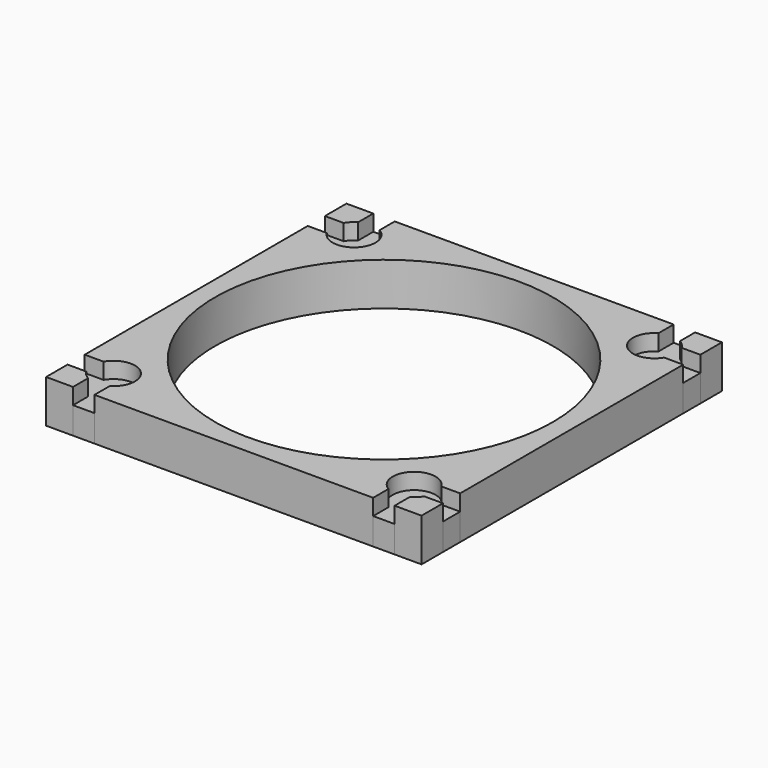
from build123d import *

# Parameters (mm, degrees)
F0_R     = 31.5
F1_DEPTH = 8
F3_DEPTH = 8
F4_DEPTH = 5
F5_DEPTH = 8
F6_DEPTH = 5


# Not quite as in the source:
# - a feature names something its author has since deleted; it is built from what else it names


with BuildPart() as f1:
    # F0 (on Top) → F1 (new body)
    with BuildSketch(Plane.XY):
        with BuildLine():
            Line((-31.4370289465, 25.9772784561), (-35, 25.9772784561))
            Line((-35, 25.9772784561), (-35, -26))
            Line((-35, -26), (-31.4875550445, -26))
            ThreePointArc((-31.4875550445, -26), (-25.2140139956, -25.1527118045), (-25.9772784561, -31.4370289465))
            Line((-25.9772784561, -31.4370289465), (-25.9772784561, -35))
            Line((-25.9772784561, -35), (25.9772784561, -35))
            Line((25.9772784561, -35), (25.9772784561, -31.4370289465))
            ThreePointArc((25.9772784561, -31.4370289465), (25.2140139956, -25.1527118045), (31.4875550445, -26))
            Line((31.4875550445, -26), (35, -26))
            Line((35, -26), (35, -25.5))
            Line((35, -25.5), (35, 25.9772784561))
            Line((35, 25.9772784561), (31.4370289465, 25.9772784561))
            ThreePointArc((31.4370289465, 25.9772784561), (25.1527118045, 25.2140139956), (26, 31.4875550445))
            Line((26, 31.4875550445), (26, 35))
            Line((26, 35), (-25.5, 35))
            Line((-25.5, 35), (-26, 35))
            Line((-26, 35), (-26, 31.4875550445))
            ThreePointArc((-26, 31.4875550445), (-25.1527118045, 25.2140139956), (-31.4370289465, 25.9772784561))
        make_face()
        Circle(F0_R, mode=Mode.SUBTRACT)
    extrude(amount=F1_DEPTH)


with BuildPart() as f3:
    # F0 (on Top) → F3 (new body)
    with BuildSketch(Plane.XY):
        with BuildLine():
            Line((-31.9894003868, 35), (-35, 35))
            Line((-35, 35), (-35, 29.9772784561))
            Line((-35, 29.9772784561), (-31.4903535301, 29.9772784561))
            ThreePointArc((-31.4903535301, 29.9772784561), (-30.8471440629, 30.83303893), (-30, 31.4875550445))
            Line((-30, 31.4875550445), (-30, 35))
            Line((-30, 35), (-30.5, 35))
            Line((-30.5, 35), (-31.9894003868, 35))
        make_face()
    extrude(amount=F3_DEPTH)


with BuildPart() as f4:
    # F0 (on Top) → F4 (new body)
    with BuildSketch(Plane.XY):
        with BuildLine():
            Line((-31.4903535301, 29.9772784561), (-35, 29.9772784561))
            Line((-35, 29.9772784561), (-35, 25.9772784561))
            Line((-35, 25.9772784561), (-31.4370289465, 25.9772784561))
            ThreePointArc((-31.4370289465, 25.9772784561), (-25.1527118045, 25.2140139956), (-26, 31.4875550445))
            Line((-26, 31.4875550445), (-26, 35))
            Line((-26, 35), (-28, 35))
            Line((-28, 35), (-30, 35))
            Line((-30, 35), (-30, 31.4875550445))
            ThreePointArc((-30, 31.4875550445), (-30.8471440629, 30.83303893), (-31.4903535301, 29.9772784561))
        make_face()
    extrude(amount=F4_DEPTH)


with BuildPart() as f5:
    # F0 (on Top) → F5 (new body)
    with BuildSketch(Plane.XY):
        with BuildLine():
            Line((29.9772784561, -31.4903535301), (29.9772784561, -35))
            Line((29.9772784561, -35), (30.5105996132, -35))
            Line((30.5105996132, -35), (35, -35))
            Line((35, -35), (35, -31.9894003868))
            Line((35, -31.9894003868), (35, -30.5))
            Line((35, -30.5), (35, -30))
            Line((35, -30), (31.4875550445, -30))
            ThreePointArc((31.4875550445, -30), (30.83303893, -30.8471440629), (29.9772784561, -31.4903535301))
        make_face()
    extrude(amount=F5_DEPTH)


with BuildPart() as f5b:
    # F0 (on Top) → F5, piece 2 (new body)
    with BuildSketch(Plane.XY):
        with BuildLine():
            Line((-31.4875550445, -30), (-35, -30))
            Line((-35, -30), (-35, -35))
            Line((-35, -35), (-29.9772784561, -35))
            Line((-29.9772784561, -35), (-29.9772784561, -31.4903535301))
            ThreePointArc((-29.9772784561, -31.4903535301), (-30.83303893, -30.8471440629), (-31.4875550445, -30))
        make_face()
    extrude(amount=F5_DEPTH)


with BuildPart() as f5c:
    # F0 (on Top) → F5, piece 3 (new body)
    with BuildSketch(Plane.XY):
        with BuildLine():
            Line((31.9894003868, 35), (30, 35))
            Line((30, 35), (30, 31.4875550445))
            ThreePointArc((30, 31.4875550445), (30.8471440629, 30.83303893), (31.4903535301, 29.9772784561))
            Line((31.4903535301, 29.9772784561), (35, 29.9772784561))
            Line((35, 29.9772784561), (35, 35))
            Line((35, 35), (31.9894003868, 35))
        make_face()
    extrude(amount=F5_DEPTH)


with BuildPart() as f6:
    # F0 (on Top) → F6 (new body)
    with BuildSketch(Plane.XY):
        with BuildLine():
            Line((25.9772784561, -31.4370289465), (25.9772784561, -35))
            Line((25.9772784561, -35), (29.9772784561, -35))
            Line((29.9772784561, -35), (29.9772784561, -31.4903535301))
            ThreePointArc((29.9772784561, -31.4903535301), (30.83303893, -30.8471440629), (31.4875550445, -30))
            Line((31.4875550445, -30), (35, -30))
            Line((35, -30), (35, -28))
            Line((35, -28), (35, -26))
            Line((35, -26), (31.4875550445, -26))
            ThreePointArc((31.4875550445, -26), (25.2140139956, -25.1527118045), (25.9772784561, -31.4370289465))
        make_face()
    extrude(amount=F6_DEPTH)


with BuildPart() as f6b:
    # F0 (on Top) → F6, piece 2 (new body)
    with BuildSketch(Plane.XY):
        with BuildLine():
            Line((-31.4875550445, -26), (-35, -26))
            Line((-35, -26), (-35, -30))
            Line((-35, -30), (-31.4875550445, -30))
            ThreePointArc((-31.4875550445, -30), (-30.83303893, -30.8471440629), (-29.9772784561, -31.4903535301))
            Line((-29.9772784561, -31.4903535301), (-29.9772784561, -35))
            Line((-29.9772784561, -35), (-25.9772784561, -35))
            Line((-25.9772784561, -35), (-25.9772784561, -31.4370289465))
            ThreePointArc((-25.9772784561, -31.4370289465), (-25.2140139956, -25.1527118045), (-31.4875550445, -26))
        make_face()
    extrude(amount=F6_DEPTH)


with BuildPart() as f6c:
    # F0 (on Top) → F6, piece 3 (new body)
    with BuildSketch(Plane.XY):
        with BuildLine():
            Line((28, 35), (26, 35))
            Line((26, 35), (26, 31.4875550445))
            ThreePointArc((26, 31.4875550445), (25.1527118045, 25.2140139956), (31.4370289465, 25.9772784561))
            Line((31.4370289465, 25.9772784561), (35, 25.9772784561))
            Line((35, 25.9772784561), (35, 29.9772784561))
            Line((35, 29.9772784561), (31.4903535301, 29.9772784561))
            ThreePointArc((31.4903535301, 29.9772784561), (30.8471440629, 30.83303893), (30, 31.4875550445))
            Line((30, 31.4875550445), (30, 35))
            Line((30, 35), (28, 35))
        make_face()
    extrude(amount=F6_DEPTH)


solid = Compound([f1.part, f3.part, f4.part, f5.part, f5b.part, f5c.part, f6.part, f6b.part, f6c.part])
